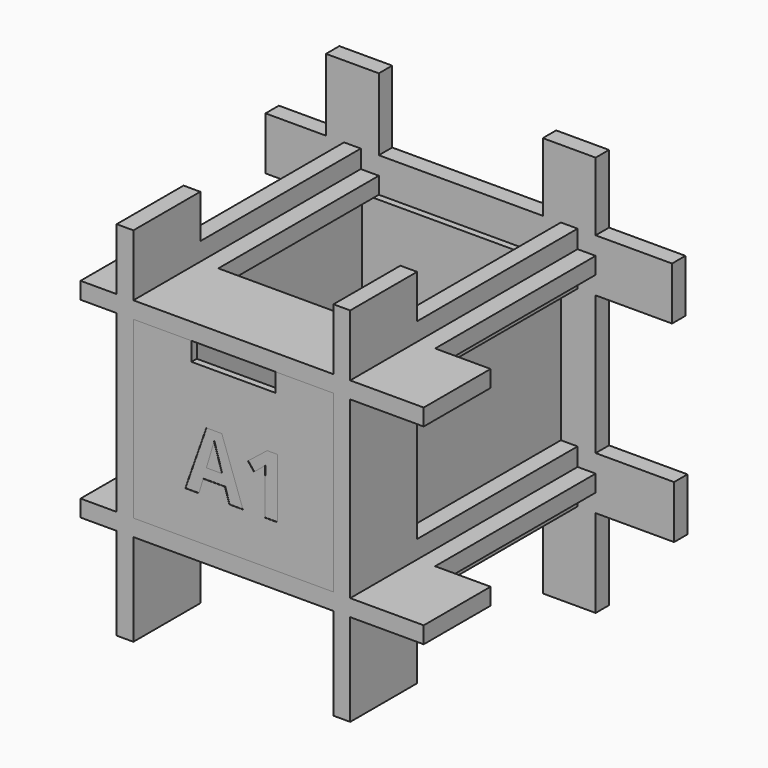
from build123d import *

# Parameters (mm, degrees)
F0_W          = 59.8487280155
F0_H          = 5
F0_W_2        = 5
F0_H_2        = 52.3382220784
F0_W_3        = 21.9838940506
F0_H_3        = 18.4198271861
F0_H_4        = 27.5841102749
F0_W_4        = 10.8073175699
F1_DEPTH      = 25
F3_DEPTH      = 60
F4_W          = 5.4036587849
F4_H          = 5.4036587849
F4_W_2        = 15.8073175699
F4_H_2        = 21.5611807629
F4_H_3        = 15.8073175699
F4_W_3        = 23.4610885908
F4_W_4        = 18.0847779289
F4_H_4        = 41.5309045086
F4_W_5        = 49.0414104457
F4_H_5        = 26.2893487519
F4_W_6        = 21.8264408782
F4_H_6        = 25.9031888848
F5_DEPTH      = 5
F6_W          = 59.8487280155
F6_H          = 52.3382220784
F7_DEPTH      = 85
F8_W          = 55.8487280155
F8_H          = 81
F9_DEPTH      = 50
F10_W         = 25.1319497978
F10_H         = 5.5549301952
F11_DEPTH     = 2
F12_TEXT_SIZE = 25.0334980794
F13_DEPTH     = 0.1


# Not quite as in the source:
# - Text() gives the source's letters only with a copy of the font that has no kerning and outlines rounded to 1/6400 em; it was checked with that copy


with BuildPart() as f1:
    # F0 (on Front) → F1 (new body)
    with BuildSketch(Plane.XZ):
        with Locations((2.9650360269, 32.9545786977)):
            Rectangle(F0_W, F0_H)
        with Locations((35.3894000346, 32.9545786977)):
            Rectangle(F0_W_2, F0_H)
        with Locations((35.3894000346, 4.2854676585)):
            Rectangle(F0_W_2, F0_H_2)
        with Locations((-29.4593279809, 32.9545786977)):
            Rectangle(F0_W_2, F0_H)
        with Locations((-29.4593279809, 4.2854676585)):
            Rectangle(F0_W_2, F0_H_2)
        with Locations((-29.4593279809, -24.3836433807)):
            Rectangle(F0_W_2, F0_H)
        with Locations((2.9650360269, -24.3836433807)):
            Rectangle(F0_W, F0_H)
        with Locations((35.3894000346, -24.3836433807)):
            Rectangle(F0_W_2, F0_H)
        with Locations((48.8813470599, 32.9545786977)):
            Rectangle(F0_W_3, F0_H)
        with Locations((35.3894000346, 44.6644922908)):
            Rectangle(F0_W_2, F0_H_3)
        with Locations((48.8813470599, -24.3836433807)):
            Rectangle(F0_W_3, F0_H)
        with Locations((35.3894000346, -40.6756985182)):
            Rectangle(F0_W_2, F0_H_4)
        with Locations((-29.4593279809, -40.6756985182)):
            Rectangle(F0_W_2, F0_H_4)
        with Locations((-37.3629867658, -24.3836433807)):
            Rectangle(F0_W_4, F0_H)
        with Locations((-37.3629867658, 32.9545786977)):
            Rectangle(F0_W_4, F0_H)
        with Locations((-29.4593279809, 44.6644922908)):
            Rectangle(F0_W_2, F0_H_3)
    extrude(amount=F1_DEPTH)

    # F2 (on face) → F3 (join)
    with BuildSketch(Plane(origin=(0, 0, 0), x_dir=(-1, 0, 0), z_dir=(0, 1, 0))):
        Polygon((-32.8894000346, 40.8582374826), (-37.8894000346, 40.8582374826), (-37.8894000346, 35.4545786977), (-43.2930588196, 35.4545786977), (-43.2930588196, 30.4545786977), (-37.8894000346, 30.4545786977), (-37.8894000346, 25.0509199128), (-32.8894000346, 25.0509199128), (-32.8894000346, 30.4545786977), (-27.4857412497, 30.4545786977), (-27.4857412497, 35.4545786977), (-32.8894000346, 35.4545786977), align=None)
        Polygon((26.9593279809, 35.4545786977), (21.5556691959, 35.4545786977), (21.5556691959, 30.4545786977), (26.9593279809, 30.4545786977), (26.9593279809, 25.0509199128), (31.9593279809, 25.0509199128), (31.9593279809, 30.4545786977), (37.3629867658, 30.4545786977), (37.3629867658, 35.4545786977), (31.9593279809, 35.4545786977), (31.9593279809, 40.8582374826), (26.9593279809, 40.8582374826), align=None)
        Polygon((31.9593279809, -16.4799845958), (26.9593279809, -16.4799845958), (26.9593279809, -21.8836433807), (21.5556691959, -21.8836433807), (21.5556691959, -26.8836433807), (26.9593279809, -26.8836433807), (26.9593279809, -32.2873021656), (31.9593279809, -32.2873021656), (31.9593279809, -26.8836433807), (37.3629867658, -26.8836433807), (37.3629867658, -21.8836433807), (31.9593279809, -21.8836433807), align=None)
        Polygon((-32.8894000346, -16.4799845958), (-37.8894000346, -16.4799845958), (-37.8894000346, -21.8836433807), (-43.2930588196, -21.8836433807), (-43.2930588196, -26.8836433807), (-37.8894000346, -26.8836433807), (-37.8894000346, -32.2873021656), (-32.8894000346, -32.2873021656), (-32.8894000346, -26.8836433807), (-27.4857412497, -26.8836433807), (-27.4857412497, -21.8836433807), (-32.8894000346, -21.8836433807), align=None)
    extrude(amount=F3_DEPTH)

    # F4 (on face) → F5 (join)
    with BuildSketch(Plane(origin=(0, 60, 0), x_dir=(-1, 0, 0), z_dir=(0, 1, 0))):
        Polygon((-43.2930588196, 61.3096654415), (-43.2930588196, 40.8582374826), (-37.8894000346, 40.8582374826), (-32.8894000346, 40.8582374826), (-27.4857412497, 40.8582374826), (-27.4857412497, 61.3096654415), align=None)
        with Locations((-40.5912294271, 38.1564080901)):
            Rectangle(F4_W, F4_H)
        Polygon((-43.2930588196, 35.4545786977), (-43.2930588196, 40.8582374826), (-66.1422088742, 40.8582374826), (-66.1422088742, 25.0509199128), (-43.2930588196, 25.0509199128), (-43.2930588196, 30.4545786977), align=None)
        Polygon((-32.8894000346, 40.8582374826), (-37.8894000346, 40.8582374826), (-37.8894000346, 35.4545786977), (-43.2930588196, 35.4545786977), (-43.2930588196, 30.4545786977), (-37.8894000346, 30.4545786977), (-37.8894000346, 25.0509199128), (-32.8894000346, 25.0509199128), (-32.8894000346, 30.4545786977), (-27.4857412497, 30.4545786977), (-27.4857412497, 35.4545786977), (-32.8894000346, 35.4545786977), align=None)
        with Locations((-30.1875706422, 38.1564080901)):
            Rectangle(F4_W, F4_H)
        with Locations((-40.5912294271, 27.7527493052)):
            Rectangle(F4_W, F4_H)
        Polygon((21.5556691959, 40.8582374826), (-27.4857412497, 40.8582374826), (-27.4857412497, 35.4545786977), (-27.4857412497, 30.4545786977), (-27.4857412497, 25.0509199128), (21.5556691959, 25.0509199128), align=None)
        Polygon((-37.8894000346, 25.0509199128), (-43.2930588196, 25.0509199128), (-43.2930588196, -16.4799845958), (-27.4857412497, -16.4799845958), (-27.4857412497, 25.0509199128), (-32.8894000346, 25.0509199128), align=None)
        with Locations((29.4593279809, 51.6388278641)):
            Rectangle(F4_W_2, F4_H_2)
        with Locations((29.4593279809, 32.9545786977)):
            Rectangle(F4_W_2, F4_H_3)
        with Locations((-35.3894000346, -24.3836433807)):
            Rectangle(F4_W_2, F4_H_3)
        with Locations((-55.023603115, -24.3836433807)):
            Rectangle(F4_W_3, F4_H_3)
        with Locations((-30.1875706422, 27.7527493052)):
            Rectangle(F4_W, F4_H)
        with Locations((46.4053757302, 32.9545786977)):
            Rectangle(F4_W_4, F4_H_3)
        with Locations((29.4593279809, 4.2854676585)):
            Rectangle(F4_W_2, F4_H_4)
        with Locations((-2.9650360269, -24.3836433807)):
            Rectangle(F4_W_5, F4_H_3)
        with Locations((-35.3894000346, -45.4319765416)):
            Rectangle(F4_W_2, F4_H_5)
        with Locations((29.4593279809, -24.3836433807)):
            Rectangle(F4_W_2, F4_H_3)
        with Locations((48.2762072049, -24.3836433807)):
            Rectangle(F4_W_6, F4_H_3)
        with Locations((29.4593279809, -45.2388966081)):
            Rectangle(F4_W_2, F4_H_6)
    extrude(amount=F5_DEPTH)


with BuildPart() as f7:
    # F6 (on face) → F7 (new body, through all)
    with BuildSketch(Plane.XZ.offset(25)):
        with Locations((2.9650360269, 4.2854676585)):
            Rectangle(F6_W, F6_H)
    extrude(amount=-F7_DEPTH)

    # F8 (on face) → F9 (cut)
    with BuildSketch(Plane.XY.offset(30.4545786977)):
        with Locations((2.9650360269, 17.5)):
            Rectangle(F8_W, F8_H)
    extrude(amount=-F9_DEPTH, mode=Mode.SUBTRACT)

    # F10 (on face) → F11 (cut, through all)
    with BuildSketch(Plane.XZ.offset(25)):
        with Locations((2.9650360269, 27.6771136001)):
            Rectangle(F10_W, F10_H)
    extrude(amount=-F11_DEPTH, mode=Mode.SUBTRACT)

    # F12 (on face) → F13 (cut)
    with BuildSketch(Plane.XZ.offset(25)):
        with Locations((-11.4542599767, -8.9868372306)):
            Text('A1', F12_TEXT_SIZE, font='Open Sans', font_style=FontStyle.BOLD, text_align=(TextAlign.LEFT, TextAlign.BOTTOM))
    extrude(amount=-F13_DEPTH, mode=Mode.SUBTRACT)


solid = Compound([f1.part, f7.part])
